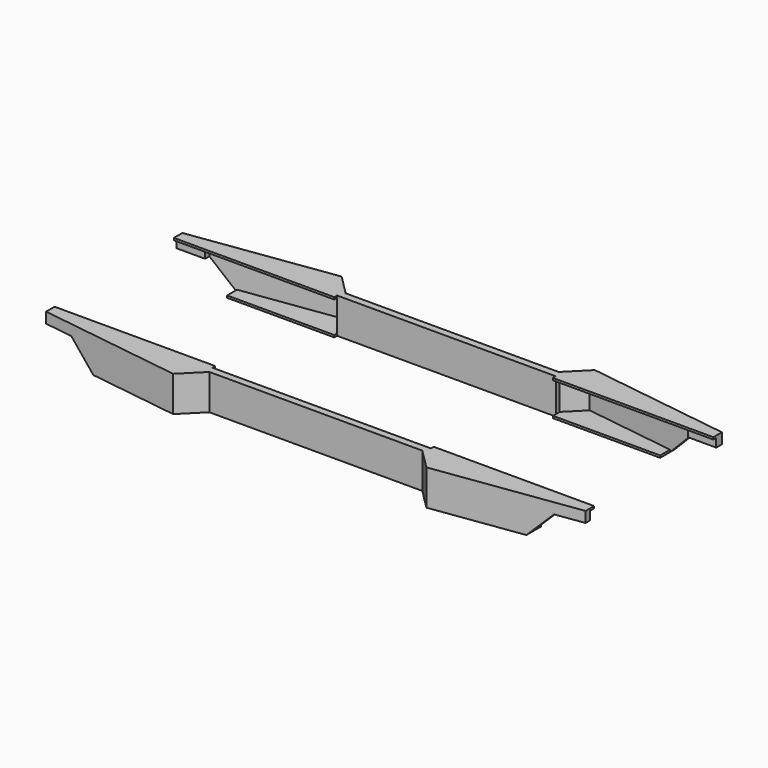
from build123d import *

# Parameters (mm, degrees)
F1_DEPTH  = 50
F3_W      = 220
F3_H      = 40
F4_DEPTH  = 760
F5_DEPTH  = 240
F6_W      = 319.9999928474
F6_H      = 220
F6_W_2    = 280
F6_H_2    = 180
F7_DEPTH  = 50
F8_DEPTH  = 435.9292732552
F9_W      = 140
F9_H      = 220
F10_DEPTH = 10
F12_DEPTH = 240
F13_DEPTH = 25
F14_DEPTH = 25
F16_W     = 220
F16_H     = 40
F17_DEPTH = 5
F15_W     = 220
F15_H     = 40
F18_DEPTH = 5
F20_DEPTH = 121.5992048383
F21_DEPTH = 1432.7406287193
F22_DEPTH = 794.6060718969
F23_DEPTH = 848.3018605039
F25_DEPTH = 50
F26_DEPTH = 50
F28_DEPTH = 50
F29_W     = 2
F29_H     = 43.9999995766
F30_DEPTH = 777.0212888718
F31_DEPTH = 308
F32_W     = 40
F32_H     = 5
F33_DEPTH = 3
F35_DEPTH = 3


# Not quite as in the source:
# - ends of sketch curves that miss each other by under 0.0002 mm in the source are joined
# - a feature names something its author has since deleted; it is built from what else it names


with BuildPart() as f1:
    # F0 (on Top) → F1 (new body)
    with BuildSketch(Plane.XY):
        Polygon((-178.3412894642, 148.3412835037), (-380, 120), (-380, -120), (-178.3412894642, -148.3412835037), (-150.0000059605, -120), (150.0000059605, -120), (178.3412894642, -148.3412835037), (380, -120), (380, 120), (178.3412894642, 148.3412835037), (150.0000059605, 120), (-150.0000059605, 120), align=None)
    extrude(amount=F1_DEPTH)

    # F3 (on face) → F4 (cut)
    with BuildSketch(Plane(origin=(-380, 0, 0), x_dir=(0, -1, 0), z_dir=(-1, 0, 0))):
        with Locations((0, 25)):
            Rectangle(F3_W, F3_H)
    extrude(amount=-F4_DEPTH, mode=Mode.SUBTRACT)

    # F2 (on face) → F5 (cut)
    with BuildSketch(Plane.XZ.offset(120)):
        Polygon((305, 0), (380, 0), (380, 35), (340, 35), align=None)
        Polygon((-340, 35), (-380, 35), (-380, 0), (-305, 0), align=None)
    extrude(amount=-F5_DEPTH, mode=Mode.SUBTRACT)

    # F6 (on face) → F7 (cut)
    with BuildSketch(Plane.XY.offset(50)):
        Rectangle(F6_W, F6_H)
        Rectangle(F6_W_2, F6_H_2, mode=Mode.SUBTRACT)
    extrude(amount=-F7_DEPTH, mode=Mode.SUBTRACT)

    # F2 (on face) → F8 (cut, symmetric)
    with BuildSketch(Plane.XZ.offset(120)):
        Polygon((-340, 35), (-380, 35), (-380, 0), (-305, 0), align=None)
        Polygon((305, 0), (380, 0), (380, 35), (340, 35), align=None)
    extrude(amount=F8_DEPTH, both=True, mode=Mode.SUBTRACT)

    # F9 (on face) → F10 (cut)
    with BuildSketch(Plane.XY.offset(50)):
        with Locations((-234.9999964237, 0)):
            Rectangle(F9_W, F9_H)
        with Locations((234.9999964237, 0)):
            Rectangle(F9_W, F9_H)
    extrude(amount=-F10_DEPTH, mode=Mode.SUBTRACT)

    # F13 (cut): a face of the model
    f13_faces = [f1.faces().sort_by_distance(p)[0] for p in [
        (0, 0, 50),
    ]]
    extrude(f13_faces, amount=-F13_DEPTH, mode=Mode.SUBTRACT)

    # F14 (cut): a face of the model
    f14_faces = [f1.faces().sort_by_distance(p)[0] for p in [
        (0, 0, 0),
    ]]
    extrude(f14_faces, amount=-F14_DEPTH, mode=Mode.SUBTRACT)

    # F16 (on face) → F17 (join)
    with BuildSketch(Plane.YZ.offset(-159.9999964237)):
        with Locations((0, 25)):
            Rectangle(F16_W, F16_H)
    extrude(amount=-F17_DEPTH)

    # F15 (on face) → F18 (join)
    with BuildSketch(Plane(origin=(159.9999964237, 0, 0), x_dir=(0, -1, 0), z_dir=(-1, 0, 0))):
        with Locations((0, 25)):
            Rectangle(F15_W, F15_H)
    extrude(amount=-F18_DEPTH)


with BuildPart() as f12:
    # F11 (on face) → F12 (new body)
    with BuildSketch(Plane.XZ.offset(120)):
        Polygon((-305.0000059605, 0), (-305.0000059605, 7.0710678119), (-332.9289381486, 35), (-340.0000059605, 35), align=None)
    extrude(amount=-F12_DEPTH)


with BuildPart() as f12b:
    # F11 (on face) → F12, piece 2 (new body)
    with BuildSketch(Plane.XZ.offset(120)):
        Polygon((340.0000059605, 35), (332.9289381486, 35), (305.0000059605, 7.0710678119), (305.0000059605, 0), align=None)
    extrude(amount=-F12_DEPTH)


with BuildPart() as f1_1:
    add(f1.part)

    # F19: union F12, F12b
    add(f12.part)
    add(f12b.part)

    # F20 (cut): a face of the model
    f20_faces = [f1_1.faces().sort_by_distance(p)[0] for p in [
        (-304.9999964237, 0, 47.5),
    ]]
    extrude(f20_faces, amount=-F20_DEPTH, mode=Mode.SUBTRACT)

    # F21 (cut, symmetric): a face of the model
    f21_faces = [f1_1.faces().sort_by_distance(p)[0] for p in [
        (304.9999964237, 0, 47.5),
    ]]
    extrude(f21_faces, amount=F21_DEPTH, both=True, mode=Mode.SUBTRACT)

    # F22 (cut, symmetric): a face of the model
    f22_faces = [f1_1.faces().sort_by_distance(p)[0] for p in [
        (-164.9999964237, 0, 25),
    ]]
    extrude(f22_faces, amount=F22_DEPTH, both=True, mode=Mode.SUBTRACT)

    # F23 (cut, symmetric): a face of the model
    f23_faces = [f1_1.faces().sort_by_distance(p)[0] for p in [
        (-159.9999964237, 0, 2.5),
    ]]
    extrude(f23_faces, amount=F23_DEPTH, both=True, mode=Mode.SUBTRACT)

    # F24 (on face) → F25 (cut)
    with BuildSketch(Plane(origin=(0, 0, 0), x_dir=(1, 0, 0), z_dir=(0, 0, -1))):
        Polygon((-154.0000059605, -110), (-301, -110), (-301, -123.0241053613), (-177.4578903454, -140.3868165731), (-154.0000059605, -116.9289321881), align=None)
        Polygon((301, -123.0241053613), (301, -110), (154.0000059605, -110), (154.0000059605, -116.9289321881), (177.4578903454, -140.3868165731), align=None)
    extrude(amount=-F25_DEPTH, mode=Mode.SUBTRACT)

    # F24 (on face) → F26 (cut)
    with BuildSketch(Plane(origin=(0, 0, 0), x_dir=(1, 0, 0), z_dir=(0, 0, -1))):
        Polygon((-301, 123.0241053613), (-301, 110), (-154.0000059605, 110), (-154.0000059605, 116.9289321881), (-177.4578903454, 140.3868165731), align=None)
        Polygon((154.0000059605, 116.9289321881), (154.0000059605, 110), (301, 110), (301, 123.0241053613), (177.4578903454, 140.3868165731), align=None)
    extrude(amount=-F26_DEPTH, mode=Mode.SUBTRACT)

    # F27 (on face) → F28 (cut)
    with BuildSketch(Plane.XY.offset(50)):
        Polygon((301, -110), (301, -123.0241053613), (340, -117.5430128079), (340, -110), align=None)
        Polygon((-301, -123.0241053613), (-301, -110), (-340, -110), (-340, -117.5430128079), align=None)
        Polygon((301, 110), (340, 110), (340, 117.5430128079), (301, 123.0241053613), align=None)
        Polygon((-340, 110), (-301, 110), (-301, 123.0241053613), (-340, 117.5430128079), align=None)
    extrude(amount=-F28_DEPTH, mode=Mode.SUBTRACT)

    # F29 (on face) → F30 (cut, symmetric)
    with BuildSketch(Plane.YZ.offset(154.0000059605)):
        with Locations((-111, 25.0000002117)):
            Rectangle(F29_W, F29_H)
    extrude(amount=F30_DEPTH, both=True, mode=Mode.SUBTRACT)

    # F29 (on face) → F31 (join)
    with BuildSketch(Plane.YZ.offset(154.0000059605)):
        with Locations((-111, 25.0000002117)):
            Rectangle(F29_W, F29_H)
    extrude(amount=-F31_DEPTH)

    # F32 (on face) → F33 (join)
    with BuildSketch(Plane.XY.offset(50)):
        Polygon((380, 105), (380, 110), (340, 110), (340, 117.5430128079), (177.4578903454, 140.3868165731), (154.0000059605, 116.9289321881), (154.0000059605, 110), (153.9999940395, 105), (340, 105), align=None)
        Polygon((-340, 117.5430128079), (-340, 110), (-380, 110), (-380, 105), (-340, 105), (-153.9999940395, 105), (-153.9999940395, 110), (-154.0000059605, 116.9289321881), (-177.4578903454, 140.3868165731), align=None)
        Polygon((-154.0000059605, -116.9289321881), (-154.0000059605, -110), (-154.0000059605, -105), (-340, -105), (-340, -110), (-340, -117.5430128079), (-177.4578903454, -140.3868165731), align=None)
        with Locations((-360, -107.5)):
            Rectangle(F32_W, F32_H)
        Polygon((340, -105), (154.0000059605, -105), (154.0000059605, -110), (154.0000059605, -116.9289321881), (177.4578903454, -140.3868165731), (340, -117.5430128079), (340, -110), align=None)
        with Locations((360, -107.5)):
            Rectangle(F32_W, F32_H)
    extrude(amount=-F33_DEPTH)

    # F34 (on face) → F35 (join)
    with BuildSketch(Plane(origin=(0, 0, 0), x_dir=(1, 0, 0), z_dir=(0, 0, -1))):
        Polygon((-154.0000059605, -116.9289321881), (-154.0000059605, -110), (-154.0000059605, -105), (-305, -105), (-305, -110), (-305, -122.4619420225), (-177.4578903454, -140.3868165731), align=None)
        Polygon((-305, 105), (-154.0000059605, 105), (-154.0000059605, 110), (-154.0000059605, 116.9289321881), (-177.4578903454, 140.3868165731), (-305, 122.4619420225), (-305, 110), align=None)
        Polygon((305, -105), (154.0000059605, -105), (154.0000059605, -110), (154.0000059605, -116.9289321881), (177.4578903454, -140.3868165731), (305, -122.4619420225), (305, -110), align=None)
        Polygon((154.0000059605, 110), (154.0000059605, 105), (305, 105), (305, 110), (305, 122.4619420225), (177.4578903454, 140.3868165731), (154.0000059605, 116.9289321881), align=None)
    extrude(amount=-F35_DEPTH)


solid = f1_1.part
